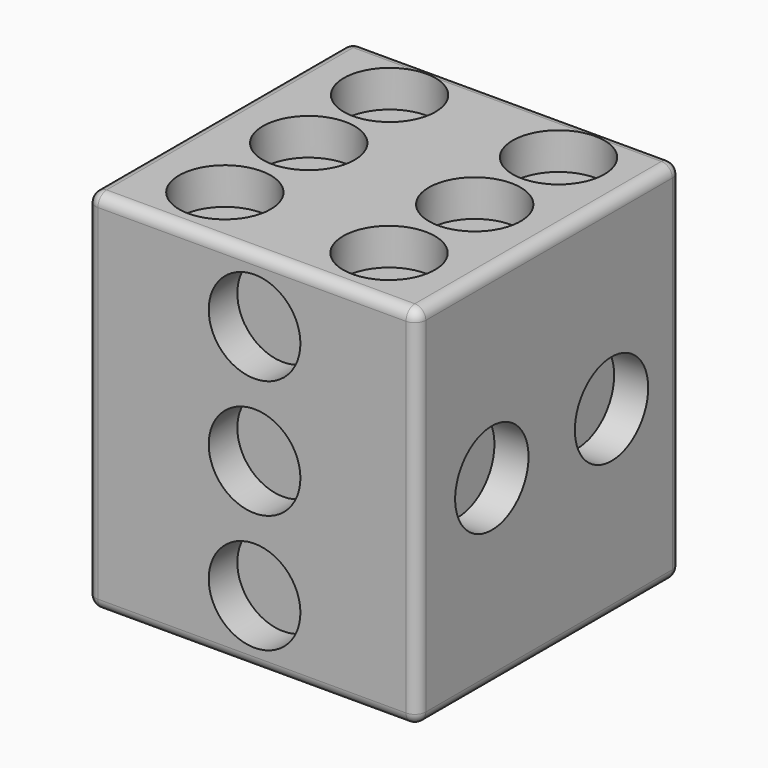
from build123d import *

# Parameters (mm, degrees)
F0_W          = 90
F0_H          = 90
F1_DEPTH      = 50
F5_R          = 12.5
F6_DEPTH      = 10
F7_R          = 12.5
F8_DEPTH      = 10
F9_R          = 12.5
F10_DEPTH     = 10
F11_R         = 12.5
F12_DEPTH     = 10
F15_R         = 12.5
F16_DEPTH     = 10
F17_R         = 12.5
F18_DEPTH     = 10
F19_R         = 12.5
F20_DEPTH     = 10
F21_R         = 12.5
F22_DEPTH     = 10
F25_R         = 12.5
F26_DEPTH     = 10
F27_R         = 12.5
F28_DEPTH     = 10
F29_R         = 12.5
F30_DEPTH     = 10
F31_T1_DEPTH  = 84
F31_T3_DEPTH  = 94
F31_T5_DEPTH  = 84
F31_S9_W      = 3
F31_S9_H      = 3
F31_T10_DEPTH = 3
F31_S15_W     = 3
F31_S15_H     = 3
F31_T16_DEPTH = 3
F31_S21_W     = 3
F31_S21_H     = 3
F31_T22_DEPTH = 3
F31_S27_W     = 3
F31_S27_H     = 3
F31_T28_DEPTH = 3
F31_S33_W     = 3
F31_S33_H     = 3
F31_T34_DEPTH = 3
F31_S39_W     = 3
F31_S39_H     = 3
F31_T40_DEPTH = 3
F31_S45_W     = 3
F31_S45_H     = 3
F31_T46_DEPTH = 3
F31_S51_W     = 3
F31_S51_H     = 3
F31_T52_DEPTH = 3


# Not quite as in the source:
# - a fillet or chamfer that OpenCascade refuses, or shapes differently, is made with other operations: its cross-section is extruded or revolved along the edge and cut away or added
# - a pattern or mirror of a feature is missing from the dataset's text; its kind, count and spacing are read off the source's solid


with BuildPart() as f1:
    # F0 (on Top) → F1 (new body)
    with BuildSketch(Plane.XY):
        with Locations((-0.7081851363, -1.7491936245)):
            Rectangle(F0_W, F0_H)
    extrude(amount=F1_DEPTH)

    # F2: F1 across plane


with BuildPart() as f1_1:
    add(f1.part)
    add(f1.part.mirror(Plane.XY))

    # F5 (on offset) → F6 (cut)
    with BuildSketch(Plane.XY.offset(-50)):
        Circle(F5_R)
    extrude(amount=F6_DEPTH, mode=Mode.SUBTRACT)

    # F7 (on offset) → F8 (cut)
    with BuildSketch(Plane.XY.offset(50)):
        with Locations((-22.6325611251, 0)):
            Circle(F7_R)
    f8 = extrude(amount=-F8_DEPTH, mode=Mode.SUBTRACT)

    # F8_copies: F8 across plane
    add(f8.mirror(Plane(origin=(0, 0, 0), x_dir=(0, 0, 1), z_dir=(1, 0, 0))), mode=Mode.SUBTRACT)

    # F9 (on offset) → F10 (cut)
    with BuildSketch(Plane.XY.offset(50)):
        with Locations((-23.0279536654, 28.0668731955)):
            Circle(F9_R)
    f10 = extrude(amount=-F10_DEPTH, mode=Mode.SUBTRACT)

    # F10_copies: F10 across plane
    add(f10.mirror(Plane(origin=(0, 0, 0), x_dir=(0, 0, 1), z_dir=(1, 0, 0))), mode=Mode.SUBTRACT)

    # F11 (on offset) → F12 (cut)
    with BuildSketch(Plane.XY.offset(50)):
        with Locations((-22.3785974085, -28.8938842714)):
            Circle(F11_R)
    f12 = extrude(amount=-F12_DEPTH, mode=Mode.SUBTRACT)

    # F12_copies: F12 across plane
    add(f12.mirror(Plane(origin=(0, 0, 0), x_dir=(0, 0, 1), z_dir=(1, 0, 0))), mode=Mode.SUBTRACT)

    # F15 (on offset) → F16 (cut)
    with BuildSketch(Plane.YZ.offset(45)):
        with Locations((-21.2455056608, 0)):
            Circle(F15_R)
    extrude(amount=-F16_DEPTH, mode=Mode.SUBTRACT)

    # F17 (on offset) → F18 (cut)
    with BuildSketch(Plane.YZ.offset(45)):
        with Locations((19.5436013028, 0)):
            Circle(F17_R)
    extrude(amount=-F18_DEPTH, mode=Mode.SUBTRACT)

    # F19 (on offset) → F20 (cut)
    with BuildSketch(Plane.YZ.offset(-46)):
        Circle(F19_R)
    extrude(amount=F20_DEPTH, mode=Mode.SUBTRACT)

    # F21 (on offset) → F22 (cut)
    with BuildSketch(Plane.YZ.offset(-46)):
        with Locations((22.0953244716, 29.4604320079)):
            Circle(F21_R)
    f22 = extrude(amount=F22_DEPTH, mode=Mode.SUBTRACT)

    # F22_copies: F22 across plane
    add(f22.mirror(Plane(origin=(0, 0, 0), x_dir=(0, -0.7999999939, 0.6000000081), z_dir=(0, -0.6000000081, -0.7999999939))), mode=Mode.SUBTRACT)

    # F22_copies1: F22 across plane
    add(f22.mirror(Plane(origin=(0, 0, 0), x_dir=(0, 0, -1), z_dir=(0, -1, 0))), mode=Mode.SUBTRACT)

    # F22_copies2: F22 across plane
    add(f22.mirror(Plane(origin=(0, 0, 0), x_dir=(-1, 0, 0), z_dir=(0, 0, -1))), mode=Mode.SUBTRACT)

    # F25 (on offset) → F26 (cut)
    with BuildSketch(Plane.XZ.offset(47)):
        Circle(F25_R)
    f26 = extrude(amount=-F26_DEPTH, mode=Mode.SUBTRACT)

    # F26_copies: F26 across plane
    add(f26.mirror(Plane(origin=(0, 0, -16.146583), x_dir=(-1, 0, 0), z_dir=(0, 0, -1))), mode=Mode.SUBTRACT)

    # F27 (on offset) → F28 (cut)
    with BuildSketch(Plane.XZ.offset(47)):
        with Locations((0, 32.2931669652)):
            Circle(F27_R)
    extrude(amount=-F28_DEPTH, mode=Mode.SUBTRACT)

    # F29 (on offset) → F30 (cut)
    with BuildSketch(Plane.XZ.offset(-44)):
        with Locations((20.3956849873, 24.9280594289)):
            Circle(F29_R)
    f30 = extrude(amount=F30_DEPTH, mode=Mode.SUBTRACT)

    # F30_copies: F30 across plane
    add(f30.mirror(Plane(origin=(0, 0, 0), x_dir=(-1, 0, 0), z_dir=(0, 0, -1))), mode=Mode.SUBTRACT)

    # F30_copies1: F30 across plane
    add(f30.mirror(Plane(origin=(0, 0, 0), x_dir=(0, 0, -1), z_dir=(-1, 0, 0))), mode=Mode.SUBTRACT)

    # F30_copies2: F30 across plane
    add(f30.mirror(Plane(origin=(0, 0, 0), x_dir=(-0.7739572992, 0, 0.6332377903), z_dir=(-0.6332377903, 0, -0.7739572992))), mode=Mode.SUBTRACT)

    # F31: fillet of radius 3 on 12 edges, made by hand

    # F31_s2 → F31_t1 (cut)
    with BuildSketch(Plane.XZ.offset(-40.2508063755)):
        with BuildLine():
            ThreePointArc((44.2918148637, 47), (43.4131352072, 49.1213203436), (41.2918148637, 50))
            Line((41.2918148637, 50), (44.2918148637, 50))
            Line((44.2918148637, 50), (44.2918148637, 47))
        make_face()
        with BuildLine():
            ThreePointArc((44.2918148637, -47), (43.4131352072, -49.1213203436), (41.2918148637, -50))
            Line((41.2918148637, -50), (44.2918148637, -50))
            Line((44.2918148637, -50), (44.2918148637, -47))
        make_face()
        with BuildLine():
            ThreePointArc((-42.7081851363, 50), (-44.8295054799, 49.1213203436), (-45.7081851363, 47))
            Line((-45.7081851363, 47), (-45.7081851363, 50))
            Line((-45.7081851363, 50), (-42.7081851363, 50))
        make_face()
        with BuildLine():
            ThreePointArc((-42.7081851363, -50), (-44.8295054799, -49.1213203436), (-45.7081851363, -47))
            Line((-45.7081851363, -47), (-45.7081851363, -50))
            Line((-45.7081851363, -50), (-42.7081851363, -50))
        make_face()
    extrude(amount=F31_T1_DEPTH, mode=Mode.SUBTRACT)

    # F31_s4 → F31_t3 (cut)
    with BuildSketch(Plane.XY.offset(-47)):
        with BuildLine():
            ThreePointArc((44.2918148637, -43.7491936245), (43.4131352072, -45.870513968), (41.2918148637, -46.7491936245))
            Line((41.2918148637, -46.7491936245), (44.2918148637, -46.7491936245))
            Line((44.2918148637, -46.7491936245), (44.2918148637, -43.7491936245))
        make_face()
        with BuildLine():
            ThreePointArc((44.2918148637, 40.2508063755), (43.4131352072, 42.3721267191), (41.2918148637, 43.2508063755))
            Line((41.2918148637, 43.2508063755), (44.2918148637, 43.2508063755))
            Line((44.2918148637, 43.2508063755), (44.2918148637, 40.2508063755))
        make_face()
        with BuildLine():
            ThreePointArc((-42.7081851363, 43.2508063755), (-44.8295054799, 42.3721267191), (-45.7081851363, 40.2508063755))
            Line((-45.7081851363, 40.2508063755), (-45.7081851363, 43.2508063755))
            Line((-45.7081851363, 43.2508063755), (-42.7081851363, 43.2508063755))
        make_face()
        with BuildLine():
            ThreePointArc((-42.7081851363, -46.7491936245), (-44.8295054799, -45.870513968), (-45.7081851363, -43.7491936245))
            Line((-45.7081851363, -43.7491936245), (-45.7081851363, -46.7491936245))
            Line((-45.7081851363, -46.7491936245), (-42.7081851363, -46.7491936245))
        make_face()
    extrude(amount=F31_T3_DEPTH, mode=Mode.SUBTRACT)

    # F31_s6 → F31_t5 (cut)
    with BuildSketch(Plane.YZ.offset(-42.7081851363)):
        with BuildLine():
            ThreePointArc((40.2508063755, -50), (42.3721267191, -49.1213203436), (43.2508063755, -47))
            Line((43.2508063755, -47), (43.2508063755, -50))
            Line((43.2508063755, -50), (40.2508063755, -50))
        make_face()
        with BuildLine():
            ThreePointArc((40.2508063755, 50), (42.3721267191, 49.1213203436), (43.2508063755, 47))
            Line((43.2508063755, 47), (43.2508063755, 50))
            Line((43.2508063755, 50), (40.2508063755, 50))
        make_face()
        with BuildLine():
            ThreePointArc((-46.7491936245, 47), (-45.870513968, 49.1213203436), (-43.7491936245, 50))
            Line((-43.7491936245, 50), (-46.7491936245, 50))
            Line((-46.7491936245, 50), (-46.7491936245, 47))
        make_face()
        with BuildLine():
            ThreePointArc((-46.7491936245, -47), (-45.870513968, -49.1213203436), (-43.7491936245, -50))
            Line((-43.7491936245, -50), (-46.7491936245, -50))
            Line((-46.7491936245, -50), (-46.7491936245, -47))
        make_face()
    extrude(amount=F31_T5_DEPTH, mode=Mode.SUBTRACT)


with BuildPart() as f31_tool8:
    # F31_s9 → F31_t10 (new body)
    with BuildSketch(Plane.YZ.offset(41.2918148637)):
        with Locations((-45.2491936245, 48.5)):
            Rectangle(F31_S9_W, F31_S9_H)
    extrude(amount=F31_T10_DEPTH)

    # F31_s11 → F31_t12 (revolve, cut)
    with BuildSketch(Plane(origin=(41.2918148637, -43.7491936245, 47), x_dir=(0, 0.7071067812, -0.7071067812), z_dir=(0, -0.7071067812, -0.7071067812))):
        with BuildLine():
            ThreePointArc((0, -3), (3, 0), (0, 3))
            Line((0, 3), (0, -3))
        make_face()
    revolve(axis=Axis((41.2918148637, -43.7491936245, 47), (1, 0, 0)), mode=Mode.SUBTRACT)


with BuildPart() as f1_2:
    add(f1_1.part)

    # F31_t7: cut F31_tool8
    add(f31_tool8.part, mode=Mode.SUBTRACT)


with BuildPart() as f31_tool14:
    # F31_s15 → F31_t16 (new body)
    with BuildSketch(Plane.YZ.offset(41.2918148637)):
        with Locations((41.7508063755, 48.5)):
            Rectangle(F31_S15_W, F31_S15_H)
    extrude(amount=F31_T16_DEPTH)

    # F31_s17 → F31_t18 (revolve, cut)
    with BuildSketch(Plane(origin=(41.2918148637, 40.2508063755, 47), x_dir=(0, -0.7071067812, -0.7071067812), z_dir=(0, -0.7071067812, 0.7071067812))):
        with BuildLine():
            ThreePointArc((0, -3), (3, 0), (0, 3))
            Line((0, 3), (0, -3))
        make_face()
    revolve(axis=Axis((41.2918148637, 40.2508063755, 47), (1, 0, 0)), mode=Mode.SUBTRACT)


with BuildPart() as f1_3:
    add(f1_2.part)

    # F31_t13: cut F31_tool14
    add(f31_tool14.part, mode=Mode.SUBTRACT)


with BuildPart() as f31_tool20:
    # F31_s21 → F31_t22 (new body)
    with BuildSketch(Plane.YZ.offset(41.2918148637)):
        with Locations((-45.2491936245, -48.5)):
            Rectangle(F31_S21_W, F31_S21_H)
    extrude(amount=F31_T22_DEPTH)

    # F31_s23 → F31_t24 (revolve, cut)
    with BuildSketch(Plane(origin=(41.2918148637, -43.7491936245, -47), x_dir=(0, 0.7071067812, 0.7071067812), z_dir=(0, 0.7071067812, -0.7071067812))):
        with BuildLine():
            ThreePointArc((0, -3), (3, 0), (0, 3))
            Line((0, 3), (0, -3))
        make_face()
    revolve(axis=Axis((41.2918148637, -43.7491936245, -47), (1, 0, 0)), mode=Mode.SUBTRACT)


with BuildPart() as f1_4:
    add(f1_3.part)

    # F31_t19: cut F31_tool20
    add(f31_tool20.part, mode=Mode.SUBTRACT)


with BuildPart() as f31_tool26:
    # F31_s27 → F31_t28 (new body)
    with BuildSketch(Plane.YZ.offset(41.2918148637)):
        with Locations((41.7508063755, -48.5)):
            Rectangle(F31_S27_W, F31_S27_H)
    extrude(amount=F31_T28_DEPTH)

    # F31_s29 → F31_t30 (revolve, cut)
    with BuildSketch(Plane(origin=(41.2918148637, 40.2508063755, -47), x_dir=(0, -0.7071067812, 0.7071067812), z_dir=(0, 0.7071067812, 0.7071067812))):
        with BuildLine():
            ThreePointArc((0, -3), (3, 0), (0, 3))
            Line((0, 3), (0, -3))
        make_face()
    revolve(axis=Axis((41.2918148637, 40.2508063755, -47), (1, 0, 0)), mode=Mode.SUBTRACT)


with BuildPart() as f1_5:
    add(f1_4.part)

    # F31_t25: cut F31_tool26
    add(f31_tool26.part, mode=Mode.SUBTRACT)


with BuildPart() as f31_tool32:
    # F31_s33 → F31_t34 (new body)
    with BuildSketch(Plane.XY.offset(-47)):
        with Locations((-44.2081851363, 41.7508063755)):
            Rectangle(F31_S33_W, F31_S33_H)
    extrude(amount=-F31_T34_DEPTH)

    # F31_s35 → F31_t36 (revolve, cut)
    with BuildSketch(Plane(origin=(-42.7081851363, 40.2508063755, -47), x_dir=(0.7071067812, -0.7071067812, 0), z_dir=(0.7071067812, 0.7071067812, 0))):
        with BuildLine():
            ThreePointArc((0, -3), (3, 0), (0, 3))
            Line((0, 3), (0, -3))
        make_face()
    revolve(axis=Axis((-42.7081851363, 40.2508063755, -47), (0, 0, -1)), mode=Mode.SUBTRACT)


with BuildPart() as f1_6:
    add(f1_5.part)

    # F31_t31: cut F31_tool32
    add(f31_tool32.part, mode=Mode.SUBTRACT)


with BuildPart() as f31_tool38:
    # F31_s39 → F31_t40 (new body)
    with BuildSketch(Plane.XY.offset(47)):
        with Locations((-44.2081851363, 41.7508063755)):
            Rectangle(F31_S39_W, F31_S39_H)
    extrude(amount=F31_T40_DEPTH)

    # F31_s41 → F31_t42 (revolve, cut)
    with BuildSketch(Plane(origin=(-42.7081851363, 40.2508063755, 47), x_dir=(0.7071067812, -0.7071067812, 0), z_dir=(-0.7071067812, -0.7071067812, 0))):
        with BuildLine():
            ThreePointArc((0, -3), (3, 0), (0, 3))
            Line((0, 3), (0, -3))
        make_face()
    revolve(axis=Axis((-42.7081851363, 40.2508063755, 47), (0, 0, 1)), mode=Mode.SUBTRACT)


with BuildPart() as f1_7:
    add(f1_6.part)

    # F31_t37: cut F31_tool38
    add(f31_tool38.part, mode=Mode.SUBTRACT)


with BuildPart() as f31_tool44:
    # F31_s45 → F31_t46 (new body)
    with BuildSketch(Plane.XZ.offset(43.7491936245)):
        with Locations((-44.2081851363, 48.5)):
            Rectangle(F31_S45_W, F31_S45_H)
    extrude(amount=F31_T46_DEPTH)

    # F31_s47 → F31_t48 (revolve, cut)
    with BuildSketch(Plane(origin=(-42.7081851363, -43.7491936245, 47), x_dir=(0.7071067812, 0, -0.7071067812), z_dir=(-0.7071067812, 0, -0.7071067812))):
        with BuildLine():
            ThreePointArc((0, -3), (3, 0), (0, 3))
            Line((0, 3), (0, -3))
        make_face()
    revolve(axis=Axis((-42.7081851363, -43.7491936245, 47), (0, -1, 0)), mode=Mode.SUBTRACT)


with BuildPart() as f1_8:
    add(f1_7.part)

    # F31_t43: cut F31_tool44
    add(f31_tool44.part, mode=Mode.SUBTRACT)


with BuildPart() as f31_tool50:
    # F31_s51 → F31_t52 (new body)
    with BuildSketch(Plane.XZ.offset(43.7491936245)):
        with Locations((-44.2081851363, -48.5)):
            Rectangle(F31_S51_W, F31_S51_H)
    extrude(amount=F31_T52_DEPTH)

    # F31_s53 → F31_t54 (revolve, cut)
    with BuildSketch(Plane(origin=(-42.7081851363, -43.7491936245, -47), x_dir=(0.7071067812, 0, 0.7071067812), z_dir=(0.7071067812, 0, -0.7071067812))):
        with BuildLine():
            ThreePointArc((0, -3), (3, 0), (0, 3))
            Line((0, 3), (0, -3))
        make_face()
    revolve(axis=Axis((-42.7081851363, -43.7491936245, -47), (0, -1, 0)), mode=Mode.SUBTRACT)


with BuildPart() as f1_9:
    add(f1_8.part)

    # F31_t49: cut F31_tool50
    add(f31_tool50.part, mode=Mode.SUBTRACT)


solid = f1_9.part
